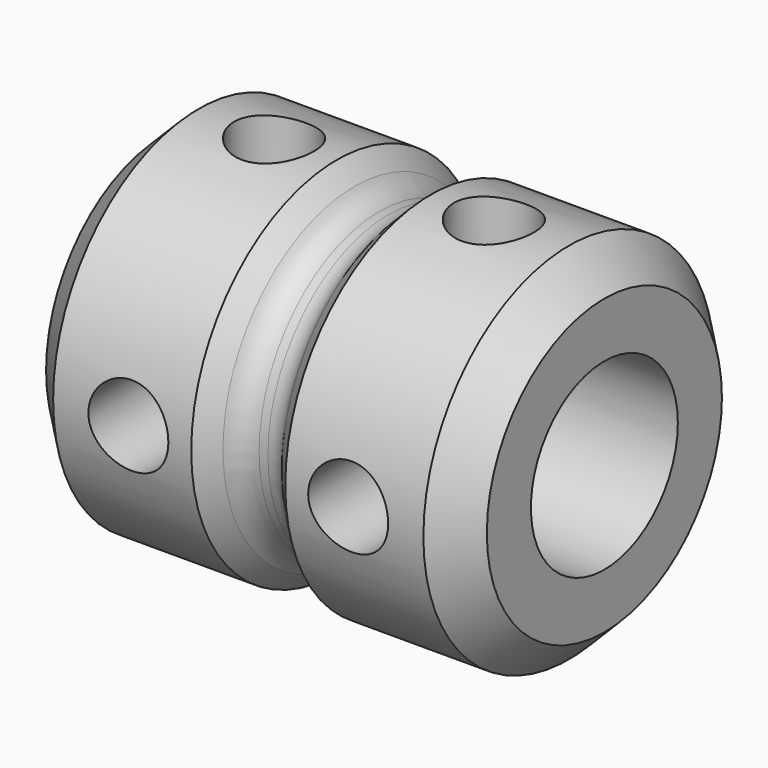
from build123d import *

# Parameters (mm, degrees)
F0_R      = 7.874
F0_R_2    = 3.96875
F1_DEPTH  = 19.05
F2_SIZE2  = 1.524
F2_SIZE   = 1.524
F5_D      = 3.4544
F5_DEPTH  = 9.49325
F5_START  = 0.9537702
F5_TIP    = 1.0378064612
F8_D      = 3.4544
F8_DEPTH  = 9.4996
F8_START  = 0.9537702
F8_TIP    = 1.0378064612
F11_SIZE2 = 0.762
F11_SIZE  = 0.762


# Not quite as in the source:
# - a fillet or chamfer that OpenCascade refuses, or shapes differently, is made with other operations: its cross-section is extruded or revolved along the edge and cut away or added


with BuildPart() as f1:
    # F0 (on Right) → F1 (new body)
    with BuildSketch(Plane.YZ):
        Circle(F0_R)
        Circle(F0_R_2, mode=Mode.SUBTRACT)
    extrude(amount=F1_DEPTH)

    # F2
    f2_edges = [f1.edges().sort_by_distance(p)[0] for p in [
        (19.05, -7.874, 0),
        (0, -7.874, 0),
    ]]
    chamfer(f2_edges, length=F2_SIZE, length2=F2_SIZE2)

    # F5
    # its depths count from where the whole tool has entered the part; down to there all is cleared
    with Locations(Plane.XY.offset(8.636).offset(-F5_START)):
        with Locations((4.7752, 0), (14.2748, 0)):
            Hole(F5_D / 2, depth=F5_DEPTH)
            with Locations((0, 0, -(F5_DEPTH + F5_TIP / 2))):  # 118° drill point
                Cone(0, F5_D / 2, F5_TIP, mode=Mode.SUBTRACT)

    # F8
    # its depths count from where the whole tool has entered the part; down to there all is cleared
    with Locations(Plane.XZ.offset(8.636).offset(-F8_START)):
        with Locations((4.7752, 0), (14.2748, 0)):
            Hole(F8_D / 2, depth=F8_DEPTH)
            with Locations((0, 0, -(F8_DEPTH + F8_TIP / 2))):  # 118° drill point
                Cone(0, F8_D / 2, F8_TIP, mode=Mode.SUBTRACT)

    # F9 (on Front) → F10 (revolve, cut)
    with BuildSketch(Plane.XZ):
        Polygon((10.795, 8.9425863698), (9.525, 8.9425863698), (8.255, 8.9425863698), (8.255, 6.5122395754), (10.795, 6.5122395754), align=None)
    revolve(axis=Axis((-2.5821820018, 0, 0), (-1, 0, 0)), mode=Mode.SUBTRACT)

    # F11
    f11_edges = [f1.edges().sort_by_distance(p)[0] for p in [
        (8.255, -7.874, 0),
        (10.795, -7.874, 0),
    ]]
    chamfer(f11_edges, length=F11_SIZE, length2=F11_SIZE2)

    # F12: fillet of radius 1.27 on 2 edges, made by hand

    # F12_s1 → F12_t2 (revolve)
    with BuildSketch(Plane.XZ):
        with BuildLine():
            ThreePointArc((8.255, 7.112), (8.7166107711, 6.6722611385), (9.3337395013, 6.5122395754))
            Line((9.3337395013, 6.5122395754), (9.3337395013, 6.4868395754))
            Line((9.3337395013, 6.4868395754), (8.255, 6.4868395754))
            Line((8.255, 6.4868395754), (8.2296, 6.5122395754))
            ThreePointArc((8.2296, 6.5122395754), (8.2296, 6.8121197877), (8.23342521, 7.0985952085))
            Line((8.23342521, 7.0985952085), (8.255, 7.112))
        make_face()
    revolve(axis=Axis((8.255, 0, 0), (-1, 0, 0)))

    # F12_s3 → F12_t4 (revolve)
    with BuildSketch(Plane.XZ):
        with BuildLine():
            ThreePointArc((9.7162604987, 6.5122395754), (10.3333892289, 6.6722611385), (10.795, 7.112))
            Line((10.795, 7.112), (10.81657479, 7.0985952085))
            ThreePointArc((10.81657479, 7.0985952085), (10.8204, 6.8121197877), (10.8204, 6.5122395754))
            Line((10.8204, 6.5122395754), (10.795, 6.4868395754))
            Line((10.795, 6.4868395754), (9.7162604987, 6.4868395754))
            Line((9.7162604987, 6.4868395754), (9.7162604987, 6.5122395754))
        make_face()
    revolve(axis=Axis((10.795, 0, 0), (-1, 0, 0)))


solid = f1.part
